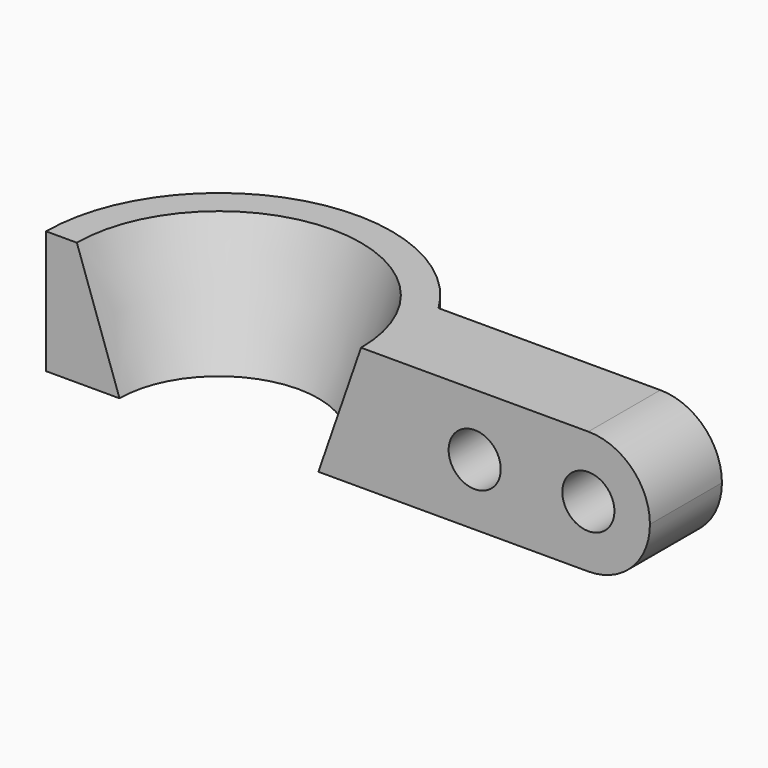
from build123d import *

# Parameters (mm, degrees)
F1_DEPTH = 52
F4_R     = 11
F5_DEPTH = 44.7
F6_R     = 25.99999


# Not quite as in the source:
# - a fillet or chamfer is up to 0.001 mm smaller than in the source, because OpenCascade refuses the exact size


with BuildPart() as f1:
    # F0 (on Top) → F1 (new body)
    with BuildSketch(Plane.XY):
        with BuildLine():
            ThreePointArc((-42, 0), (0, 42), (42, 0))
            Line((42, 0), (182, 0))
            Line((182, 0), (182, 38))
            Line((182, 38), (62.329768169, 38))
            ThreePointArc((62.329768169, 38), (-19.7348286497, 70.2818364741), (-73, 0))
            Line((-73, 0), (-42, 0))
        make_face()
    extrude(amount=F1_DEPTH)

    # F2 (on face) → F3 (revolve, cut)
    with BuildSketch(Plane.XZ):
        Polygon((0, 0), (0, 52), (-60, 52), (-42, 0), align=None)
    revolve(axis=Axis((0, 0, 26), (0, 0, -1)), mode=Mode.SUBTRACT)

    # F4 (on face) → F5 (cut)
    with BuildSketch(Plane.XZ):
        with Locations((108, 26)):
            Circle(F4_R)
        with Locations((156, 26)):
            Circle(F4_R)
    extrude(amount=-F5_DEPTH, mode=Mode.SUBTRACT)

    # F6 (radius 26 in the source; OpenCascade refuses exactly that, so slightly less here)
    f6_edges = [f1.edges().sort_by_distance(p)[0] for p in [
        (182, 19, 52),
        (182, 19, 0),
    ]]
    fillet(f6_edges, radius=F6_R)


solid = f1.part
